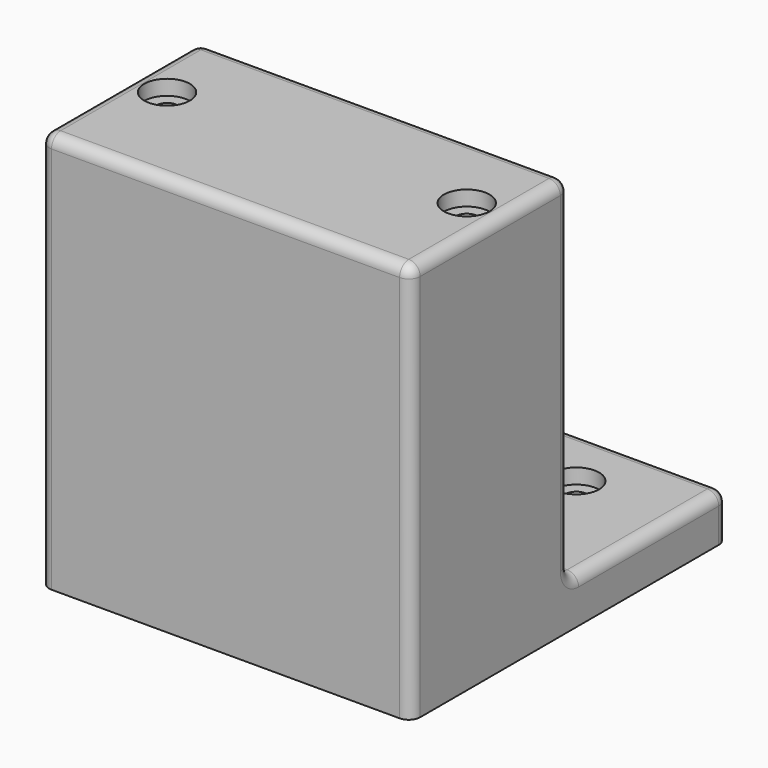
from build123d import *

# Parameters (mm, degrees)
F0_W           = 82.55
F0_H           = 88.9
F1_DEPTH       = 44.069
F2_W           = 82.55
F2_H           = 10.16
F3_DEPTH       = 44.069
F5_D           = 4.826
F5_CBORE_D     = 10.16
F5_CBORE_DEPTH = 3.3528
F6_R           = 2.54
F8_D           = 4.826
F8_CBORE_D     = 10.16
F8_CBORE_DEPTH = 3.3528


# Not quite as in the source:
# - a feature names something its author has since deleted; it is built from what else it names


with BuildPart() as f1:
    # F0 (on Front) → F1 (new body)
    with BuildSketch(Plane.XZ):
        Rectangle(F0_W, F0_H)
    extrude(amount=F1_DEPTH)

    # F2 (on face) → F3 (join)
    with BuildSketch(Plane(origin=(0, 0, 0), x_dir=(-1, 0, 0), z_dir=(0, 1, 0))):
        with Locations((0, -39.37)):
            Rectangle(F2_W, F2_H)
    extrude(amount=F3_DEPTH)

    # F5 (through all)
    with Locations(Plane.XY.offset(44.45)):
        with Locations((-33.3502, -18.669), (33.3502, -18.669)):
            CounterBoreHole(F5_D / 2, F5_CBORE_D / 2, F5_CBORE_DEPTH)

    # F6
    f6_edges = [f1.edges().sort_by_distance(p)[0] for p in [
        (-41.275, -22.0345, 44.45),
        (41.275, -22.0345, 44.45),
        (0, -44.069, 44.45),
        (0, 0, 44.45),
        (41.275, -44.069, 0),
        (41.275, 0, 5.08),
        (-41.275, -44.069, 0),
        (-41.275, 0, 5.08),
        (-41.275, 22.0345, -34.29),
        (0, 44.069, -34.29),
        (41.275, 22.0345, -34.29),
        (0, 0, -34.29),
        (41.275, 44.069, -39.37),
        (-41.275, 44.069, -39.37),
    ]]
    fillet(f6_edges, radius=F6_R)

    # F8 (through all)
    with Locations(Plane.XY.offset(-34.29)):
        with Locations((-19.1008, 29.6364016831), (19.0881, 29.6364016831)):
            CounterBoreHole(F8_D / 2, F8_CBORE_D / 2, F8_CBORE_DEPTH)


solid = f1.part
